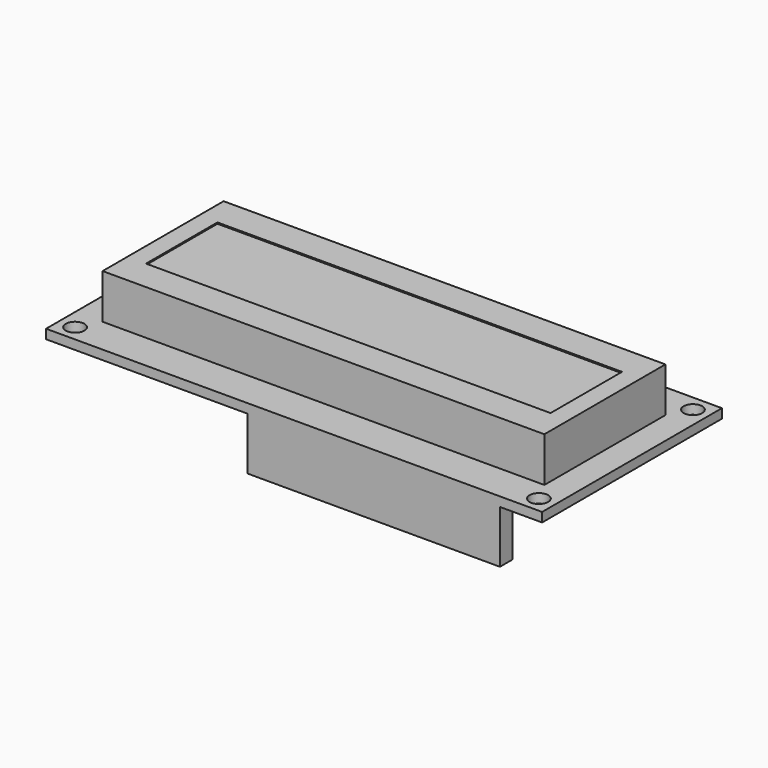
from build123d import *

# Parameters (mm, degrees)
F0_W        = 71.25
F0_H        = 24.4
F0_W_2      = 65.25
F0_H_2      = 14.4
F1_DEPTH    = 7
F2_DEPTH    = 7.2
F3_W        = 17.4
F3_H        = 2.85
F4_DEPTH    = 3.75
F5_T4_DEPTH = 23.4234639037
F5_T9_DEPTH = 23.4234639037
F6_W        = 80
F6_H        = 36.25
F6_R        = 1.5
F7_DEPTH    = 1.5
F8_W        = 40.7
F8_H        = 2.5
F9_DEPTH    = 8.5


# Not quite as in the source:
# - a fillet or chamfer that OpenCascade refuses, or shapes differently, is made with other operations: its cross-section is extruded or revolved along the edge and cut away or added


with BuildPart() as f1:
    # F0 (on Top) → F1 (new body)
    with BuildSketch(Plane.XY):
        Rectangle(F0_W, F0_H)
        Rectangle(F0_W_2, F0_H_2, mode=Mode.SUBTRACT)
        Rectangle(F0_W_2, F0_H_2)
    extrude(amount=F1_DEPTH)

    # F0 (on Top) → F2 (join)
    with BuildSketch(Plane.XY):
        Rectangle(F0_W, F0_H)
        Rectangle(F0_W_2, F0_H_2, mode=Mode.SUBTRACT)
    extrude(amount=F2_DEPTH)

    # F3 (on face) → F4 (join)
    with BuildSketch(Plane(origin=(-35.625, 0, 0), x_dir=(0, -1, 0), z_dir=(-1, 0, 0))):
        with Locations((0, 1.425)):
            Rectangle(F3_W, F3_H)
    extrude(amount=F4_DEPTH)

    # F5: chamfer of 4 on 2 edges, made by hand


with BuildPart() as f5_tool2:
    # F5_s3 → F5_t4 (new body)
    with BuildSketch(Plane.XY.offset(-10.2867319519)):
        Polygon((-35.375, -8.7), (-39.375, -4.7), (-39.375, -8.7), align=None)
    extrude(amount=F5_T4_DEPTH)

    split(bisect_by=Plane.YZ.offset(-35.625), keep=Keep.BOTTOM)


with BuildPart() as f1_1:
    add(f1.part)

    # F5_t1: cut F5_tool2
    add(f5_tool2.part, mode=Mode.SUBTRACT)


with BuildPart() as f5_tool7:
    # F5_s8 → F5_t9 (new body)
    with BuildSketch(Plane.XY.offset(13.1367319519)):
        Polygon((-35.375, 8.7), (-39.375, 4.7), (-39.375, 8.7), align=None)
    extrude(amount=-F5_T9_DEPTH)

    split(bisect_by=Plane.YZ.offset(-35.625), keep=Keep.BOTTOM)


with BuildPart() as f1_2:
    add(f1_1.part)

    # F5_t6: cut F5_tool7
    add(f5_tool7.part, mode=Mode.SUBTRACT)

    # F6 (on Top) → F7 (join)
    with BuildSketch(Plane.XY):
        Rectangle(F6_W, F6_H)
        with Locations((-37.4, -15.525)):
            Circle(F6_R, mode=Mode.SUBTRACT)
        with Locations((37.4, -15.525)):
            Circle(F6_R, mode=Mode.SUBTRACT)
        with Locations((-37.4, 15.525)):
            Circle(F6_R, mode=Mode.SUBTRACT)
        with Locations((37.4, 15.525)):
            Circle(F6_R, mode=Mode.SUBTRACT)
    extrude(amount=-F7_DEPTH)

    # F8 (on face) → F9 (join)
    with BuildSketch(Plane(origin=(0, 0, -1.5), x_dir=(1, 0, 0), z_dir=(0, 0, -1))):
        with Locations((12.85, 16.875)):
            Rectangle(F8_W, F8_H)
    extrude(amount=F9_DEPTH)


solid = f1_2.part
